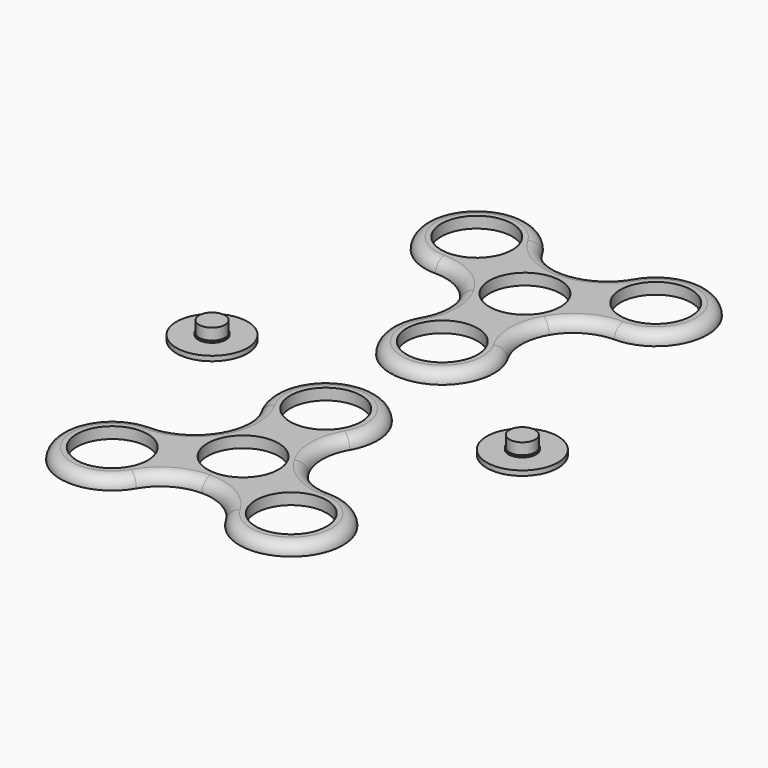
from build123d import *

# Parameters (mm, degrees)
F0_R     = 10.9897597756
F1_DEPTH = 3.5
F2_R     = 3.49999
F3_R     = 11
F3_R_2   = 4.25
F4_DEPTH = 1.5
F3_R_3   = 4
F5_DEPTH = 2
F6_DEPTH = 5.5


# Not quite as in the source:
# - a fillet or chamfer is up to 0.001 mm smaller than in the source, because OpenCascade refuses the exact size
# - a feature names something its author has since deleted; it is built from what else it names


with BuildPart() as f1:
    # F0 (on Top) → F1 (new body)
    with BuildSketch(Plane.XY):
        with BuildLine():
            ThreePointArc((-13.8435071231, -23.9776576922), (-7.9925525641, -18.1267031332), (0, -15.9851051281))
            ThreePointArc((0, -15.9851051281), (7.9925525641, -18.1267031332), (13.8435071231, -23.9776576922))
            ThreePointArc((13.8435071231, -23.9776576922), (41.5305213694, -23.9776576922), (27.6870142463, 0))
            ThreePointArc((27.6870142463, 0), (19.6944616822, 2.141598005), (13.8435071231, 7.9925525641))
            ThreePointArc((13.8435071231, 7.9925525641), (11.7019091181, 15.9851051281), (13.8435071231, 23.9776576922))
            ThreePointArc((13.8435071231, 23.9776576922), (0, 47.9553153844), (-13.8435071231, 23.9776576922))
            ThreePointArc((-13.8435071231, 23.9776576922), (-11.7019091181, 15.9851051281), (-13.8435071231, 7.9925525641))
            ThreePointArc((-13.8435071231, 7.9925525641), (-19.6944616822, 2.141598005), (-27.6870142463, 0))
            ThreePointArc((-27.6870142463, 0), (-41.5305213694, -23.9776576922), (-13.8435071231, -23.9776576922))
        make_face()
        with Locations((-27.6870142463, -15.9851051281)):
            Circle(F0_R, mode=Mode.SUBTRACT)
        Circle(F0_R, mode=Mode.SUBTRACT)
        with Locations((27.6870142463, -15.9851051281)):
            Circle(F0_R, mode=Mode.SUBTRACT)
        with Locations((0, 31.9702102563)):
            Circle(F0_R, mode=Mode.SUBTRACT)
    extrude(amount=F1_DEPTH)

    # F2 (radius 3.5 in the source; OpenCascade refuses exactly that, so slightly less here)
    f2_edges = [f1.edges().sort_by_distance(p)[0] for p in [
        (-41.530521, -23.977658, 3.5),
        (0, 47.955315, 3.5),
        (-13.843507, 7.992553, 3.5),
        (0, -15.985105, 3.5),
        (41.530521, -23.977658, 3.5),
        (13.843507, 7.992553, 3.5),
    ]]
    fillet(f2_edges, radius=F2_R)


with BuildPart() as f4:
    # F3 (on Top) → F4 (new body)
    with BuildSketch(Plane.XY):
        with Locations((-48, 48)):
            Circle(F3_R)
        with Locations((-48, 48)):
            Circle(F3_R_2, mode=Mode.SUBTRACT)
    extrude(amount=F4_DEPTH)

    # F3 (on Top) → F5 (join)
    with BuildSketch(Plane.XY):
        with Locations((-48, 48)):
            Circle(F3_R_2)
        with Locations((-48, 48)):
            Circle(F3_R_3, mode=Mode.SUBTRACT)
    extrude(amount=F5_DEPTH)

    # F3 (on Top) → F6 (join)
    with BuildSketch(Plane.XY):
        with Locations((-48, 48)):
            Circle(F3_R_3)
    extrude(amount=F6_DEPTH)


with BuildPart() as f4b:
    # F3 (on Top) → F4, piece 2 (new body)
    with BuildSketch(Plane.XY):
        with Locations((48, 48)):
            Circle(F3_R)
        with Locations((48, 48)):
            Circle(F3_R_2, mode=Mode.SUBTRACT)
    extrude(amount=F4_DEPTH)

    # F3 (on Top) → F5, piece 2 (join)
    with BuildSketch(Plane.XY):
        with Locations((48, 48)):
            Circle(F3_R_2)
        with Locations((48, 48)):
            Circle(F3_R_3, mode=Mode.SUBTRACT)
    extrude(amount=F5_DEPTH)

    # F3 (on Top) → F6, piece 2 (join)
    with BuildSketch(Plane.XY):
        with Locations((48, 48)):
            Circle(F3_R_3)
    extrude(amount=F6_DEPTH)


with BuildPart() as f7_1:
    # F7: instance of F1
    add(f1.part.mirror(Plane.XZ))


with BuildPart() as f7_1_1:
    # F8: moved
    add(f7_1.part.moved(Location((0, 109, 0))))


solid = Compound([f1.part, f4.part, f4b.part, f7_1_1.part])
